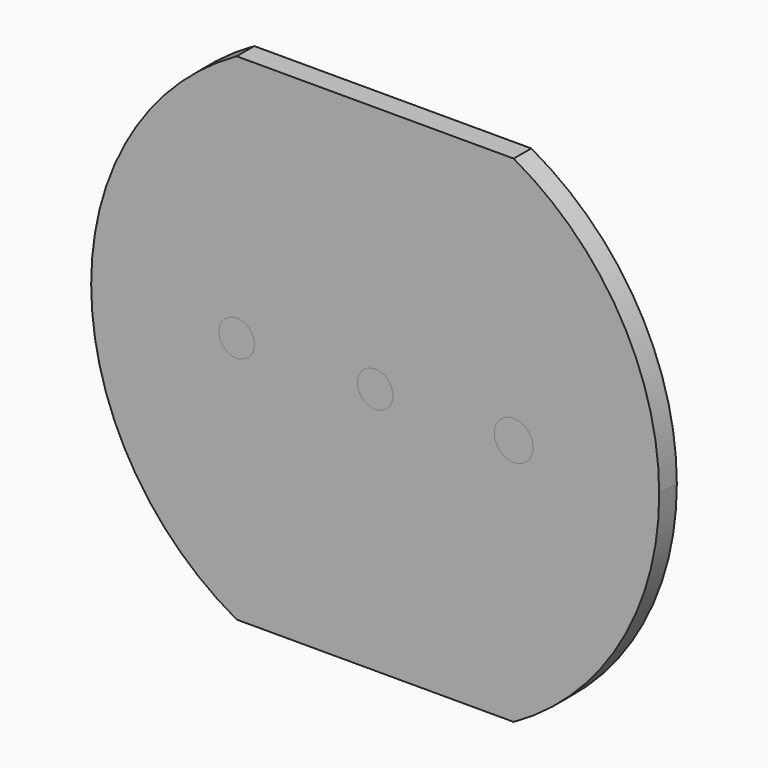
from build123d import *

# Parameters (mm, degrees)
F8_DEPTH = 7.5


# Not quite as in the source:
# - a feature of the source that left no trace in its solid (it failed there, or was rolled back) is left out
# - a feature names something its author has since deleted; it is built from what else it names


with BuildPart() as f3:
    # F2 (on Right) → F3 (revolve)
    with BuildSketch(Plane.YZ):
        with BuildLine():
            Line((0, 0), (5, 0))
            Line((5, 0), (40, 0))
            Line((40, 0), (40, 2.5))
            Line((40, 2.5), (8.8, 2.5))
            ThreePointArc((8.8, 2.5), (8.2343145751, 2.7343145751), (8, 3.3))
            Line((8, 3.3), (8, 4.4213395849))
            ThreePointArc((8, 4.4213395849), (7.7656854249, 4.9870250099), (7.2, 5.2213395849))
            Line((7.2, 5.2213395849), (2.9166693582, 5.2213395849))
            ThreePointArc((2.9166693582, 5.2213395849), (2.3761971921, 5.4315177155), (2.1197135998, 5.9516149907))
            Line((2.1197135998, 5.9516149907), (1, 18.75))
            Line((1, 18.75), (0, 18.75))
            Line((0, 18.75), (0, 5.2213395849))
            Line((0, 5.2213395849), (0, 0))
        make_face()
    revolve(axis=Axis((0, 20, 0), (0, 1, 0)))


with BuildPart() as f5_1:
    # F5: copy of F3
    add(f3.part.moved(Location((-47.1589879045, 0, -0.0356367438))))


with BuildPart() as f6_1:
    # F6: copy of F3
    add(f3.part.moved(Location((47.1589879045, 0, -0.0356367438))))


with BuildPart() as f8:
    # F7 (on Front) → F8 (new body)
    with BuildSketch(Plane.XZ):
        with BuildLine():
            Line((-53.1802220321, 0), (-96.7034770935, 0))
            ThreePointArc((-96.7034770935, 0), (-83.4026396122, -48.9444806664), (-47.1589879045, -84.4250693917))
            Line((-47.1589879045, -84.4250693917), (47.1589879045, -84.4250693917))
            ThreePointArc((47.1589879045, -84.4250693917), (83.4026396122, -48.9444806664), (96.7034770935, 0))
            Line((96.7034770935, 0), (53.7821824012, 0))
            ThreePointArc((53.7821824012, 0), (53.7822543057, -0.0178183074), (53.782278274, -0.0356367438))
            ThreePointArc((53.782278274, -0.0356367438), (47.1411694682, -6.658903145), (40.5357934079, 0))
            Line((40.5357934079, 0), (6.0394279868, 0))
            ThreePointArc((6.0394279868, 0), (0, -6.0394279868), (-6.0394279868, 0))
            Line((-6.0394279868, 0), (-41.1377537769, 0))
            ThreePointArc((-41.1377537769, 0), (-41.137674684, -0.0178182939), (-41.1376483196, -0.0356367438))
            ThreePointArc((-41.1376483196, -0.0356367438), (-47.1768063545, -6.0569499643), (-53.1802220321, 0))
        make_face()
        with BuildLine():
            Line((47.1589879045, 84.4250693917), (-47.1589879045, 84.4250693917))
            ThreePointArc((-47.1589879045, 84.4250693917), (-83.4026396122, 48.9444806664), (-96.7034770935, 0))
            Line((-96.7034770935, 0), (-53.1802220321, 0))
            ThreePointArc((-53.1802220321, 0), (-47.1589879045, 5.9857028411), (-41.1377537769, 0))
            Line((-41.1377537769, 0), (-6.0394279868, 0))
            ThreePointArc((-6.0394279868, 0), (0, 6.0394279868), (6.0394279868, 0))
            Line((6.0394279868, 0), (40.5357934079, 0))
            ThreePointArc((40.5357934079, 0), (47.1589879045, 6.5876536256), (53.7821824012, 0))
            Line((53.7821824012, 0), (96.7034770935, 0))
            ThreePointArc((96.7034770935, 0), (83.4026396122, 48.9444806664), (47.1589879045, 84.4250693917))
        make_face()
    extrude(amount=-F8_DEPTH)


solid = Compound([f3.part, f5_1.part, f6_1.part, f8.part])
